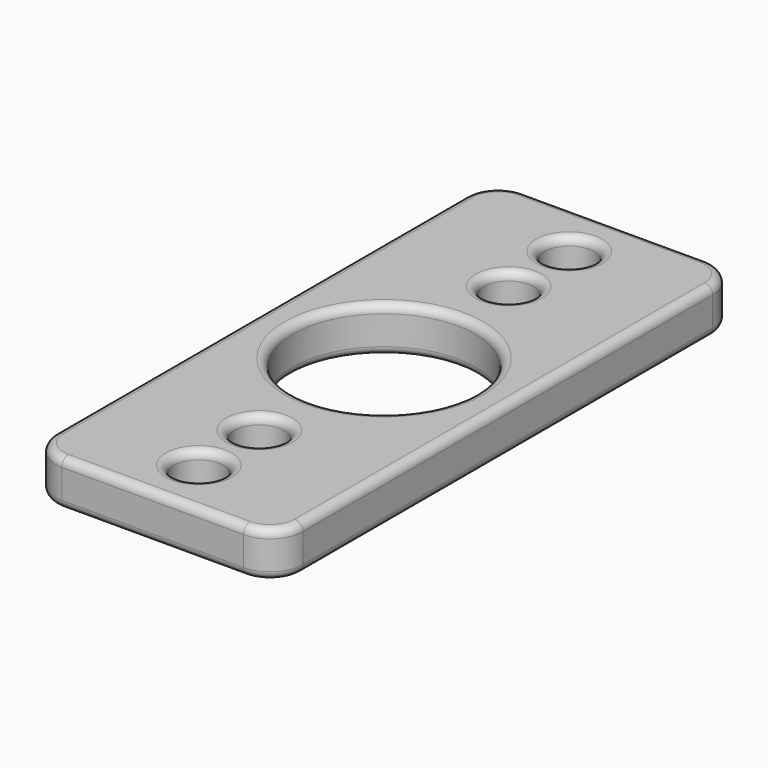
from build123d import *

# Parameters (mm, degrees)
F0_W         = 30
F0_H         = 70
F0_R         = 3
F0_R_2       = 11.025
F1_DEPTH     = 5.5
F2_R         = 1
F3_T1_DEPTH  = 5.5
F3_T4_ANGLE  = 90
F3_T6_ANGLE  = 90
F3_T8_ANGLE  = 90
F3_T10_ANGLE = 90
F3_T12_ANGLE = 90
F3_T14_ANGLE = 90
F3_T16_ANGLE = 90
F3_T18_ANGLE = 90


# Not quite as in the source:
# - a fillet or chamfer that OpenCascade refuses, or shapes differently, is made with other operations: its cross-section is extruded or revolved along the edge and cut away or added


with BuildPart() as f1:
    # F0 (on Top) → F1 (new body)
    with BuildSketch(Plane.XY):
        Rectangle(F0_W, F0_H)
        with Locations((0, -28.0352663249)):
            Circle(F0_R, mode=Mode.SUBTRACT)
        with Locations((0, -18.8642609864)):
            Circle(F0_R, mode=Mode.SUBTRACT)
        Circle(F0_R_2, mode=Mode.SUBTRACT)
        with Locations((0, 18.8642609864)):
            Circle(F0_R, mode=Mode.SUBTRACT)
        with Locations((0, 28.0352663249)):
            Circle(F0_R, mode=Mode.SUBTRACT)
    extrude(amount=F1_DEPTH)

    # F2
    f2_edges = [f1.edges().sort_by_distance(p)[0] for p in [
        (15, 0, 5.5),
        (0, 35, 5.5),
        (-15, 0, 5.5),
        (0, -35, 5.5),
        (-3, -28.035266, 5.5),
        (-3, -18.864261, 5.5),
        (-11.025, 0, 5.5),
        (-3, 18.864261, 5.5),
        (-3, 28.035266, 5.5),
        (15, 0, 0),
        (0, 35, 0),
        (-15, 0, 0),
        (0, -35, 0),
        (-3, -28.035266, 0),
        (-3, -18.864261, 0),
        (-11.025, 0, 0),
        (-3, 18.864261, 0),
        (-3, 28.035266, 0),
    ]]
    fillet(f2_edges, radius=F2_R)

    # F3: fillet of radius 4 on 4 edges, made by hand

    # F3_s2 → F3_t1 (cut)
    with BuildSketch(Plane.XY):
        with BuildLine():
            ThreePointArc((-11, -35), (-13.8284271247, -33.8284271247), (-15, -31))
            Line((-15, -31), (-15, -35))
            Line((-15, -35), (-11, -35))
        make_face()
        with BuildLine():
            ThreePointArc((15, -31), (13.8284271247, -33.8284271247), (11, -35))
            Line((11, -35), (15, -35))
            Line((15, -35), (15, -31))
        make_face()
        with BuildLine():
            ThreePointArc((15, 31), (13.8284271247, 33.8284271247), (11, 35))
            Line((11, 35), (15, 35))
            Line((15, 35), (15, 31))
        make_face()
        with BuildLine():
            ThreePointArc((-11, 35), (-13.8284271247, 33.8284271247), (-15, 31))
            Line((-15, 31), (-15, 35))
            Line((-15, 35), (-11, 35))
        make_face()
    extrude(amount=F3_T1_DEPTH, mode=Mode.SUBTRACT)

    # F3_s3 → F3_t4 (revolve, cut)
    with BuildSketch(Plane.XZ.offset(-31)):
        with BuildLine():
            ThreePointArc((-14, 0), (-14.7071067812, 0.2928932188), (-15, 1))
            Line((-15, 1), (-15, 0))
            Line((-15, 0), (-14, 0))
        make_face()
    revolve(axis=Axis((-11, 31, 0), (0, 0, -1)), revolution_arc=F3_T4_ANGLE, mode=Mode.SUBTRACT)

    # F3_s5 → F3_t6 (revolve, cut)
    with BuildSketch(Plane.YZ.offset(-11)):
        with BuildLine():
            ThreePointArc((34, 5.5), (34.7071067812, 5.2071067812), (35, 4.5))
            Line((35, 4.5), (35, 5.5))
            Line((35, 5.5), (34, 5.5))
        make_face()
    revolve(axis=Axis((-11, 31, 5.5), (0, 0, 1)), revolution_arc=F3_T6_ANGLE, mode=Mode.SUBTRACT)

    # F3_s7 → F3_t8 (revolve, cut)
    with BuildSketch(Plane.YZ.offset(11)):
        with BuildLine():
            ThreePointArc((34, 0), (34.7071067812, 0.2928932188), (35, 1))
            Line((35, 1), (35, 0))
            Line((35, 0), (34, 0))
        make_face()
    revolve(axis=Axis((11, 31, 0), (0, 0, -1)), revolution_arc=F3_T8_ANGLE, mode=Mode.SUBTRACT)

    # F3_s9 → F3_t10 (revolve, cut)
    with BuildSketch(Plane.XZ.offset(-31)):
        with BuildLine():
            ThreePointArc((14, 5.5), (14.7071067812, 5.2071067812), (15, 4.5))
            Line((15, 4.5), (15, 5.5))
            Line((15, 5.5), (14, 5.5))
        make_face()
    revolve(axis=Axis((11, 31, 5.5), (0, 0, 1)), revolution_arc=F3_T10_ANGLE, mode=Mode.SUBTRACT)

    # F3_s11 → F3_t12 (revolve, cut)
    with BuildSketch(Plane.XZ.offset(31)):
        with BuildLine():
            ThreePointArc((14, 0), (14.7071067812, 0.2928932188), (15, 1))
            Line((15, 1), (15, 0))
            Line((15, 0), (14, 0))
        make_face()
    revolve(axis=Axis((11, -31, 0), (0, 0, -1)), revolution_arc=F3_T12_ANGLE, mode=Mode.SUBTRACT)

    # F3_s13 → F3_t14 (revolve, cut)
    with BuildSketch(Plane.YZ.offset(11)):
        with BuildLine():
            ThreePointArc((-34, 5.5), (-34.7071067812, 5.2071067812), (-35, 4.5))
            Line((-35, 4.5), (-35, 5.5))
            Line((-35, 5.5), (-34, 5.5))
        make_face()
    revolve(axis=Axis((11, -31, 5.5), (0, 0, 1)), revolution_arc=F3_T14_ANGLE, mode=Mode.SUBTRACT)

    # F3_s15 → F3_t16 (revolve, cut)
    with BuildSketch(Plane.YZ.offset(-11)):
        with BuildLine():
            ThreePointArc((-34, 0), (-34.7071067812, 0.2928932188), (-35, 1))
            Line((-35, 1), (-35, 0))
            Line((-35, 0), (-34, 0))
        make_face()
    revolve(axis=Axis((-11, -31, 0), (0, 0, -1)), revolution_arc=F3_T16_ANGLE, mode=Mode.SUBTRACT)

    # F3_s17 → F3_t18 (revolve, cut)
    with BuildSketch(Plane.XZ.offset(31)):
        with BuildLine():
            ThreePointArc((-14, 5.5), (-14.7071067812, 5.2071067812), (-15, 4.5))
            Line((-15, 4.5), (-15, 5.5))
            Line((-15, 5.5), (-14, 5.5))
        make_face()
    revolve(axis=Axis((-11, -31, 5.5), (0, 0, 1)), revolution_arc=F3_T18_ANGLE, mode=Mode.SUBTRACT)


solid = f1.part
